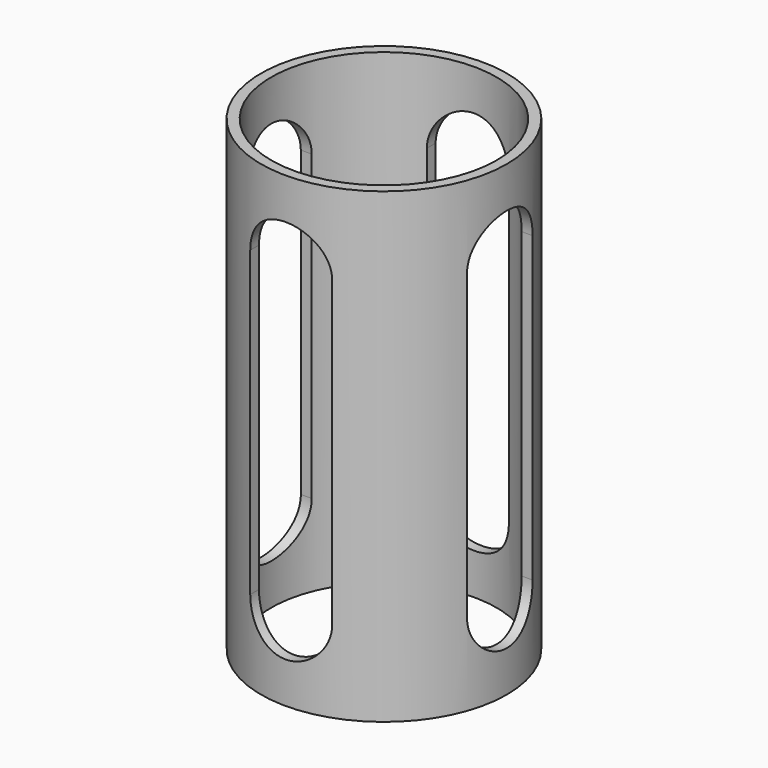
from build123d import *

# Parameters (mm, degrees)
F0_R            = 19.05
F0_R_2          = 17.4625
F1_DEPTH        = 72.39
F3_DEPTH        = 25.4
F3_COPIES_COUNT = 4


# Not quite as in the source:
# - a pattern or mirror of a feature is missing from the dataset's text; its kind, count and spacing are read off the source's solid


with BuildPart() as f1:
    # F0 (on Top) → F1 (new body)
    with BuildSketch(Plane.XY):
        Circle(F0_R)
        Circle(F0_R_2, mode=Mode.SUBTRACT)
    extrude(amount=F1_DEPTH)

    # F2 (on Front) → F3 (cut)
    with BuildSketch(Plane.XZ):
        with BuildLine():
            Line((-6.35, 59.69), (-6.35, 12.7))
            ThreePointArc((-6.35, 12.7), (0, 6.35), (6.35, 12.7))
            Line((6.35, 12.7), (6.35, 59.69))
            ThreePointArc((6.35, 59.69), (0, 66.04), (-6.35, 59.69))
        make_face()
    f3 = extrude(amount=-F3_DEPTH, mode=Mode.SUBTRACT)

    # F3_copies: F3 ×4 about axis
    f3_copies_axis = Axis((0, 0, 0), (0, 0, 1))
    for i in range(1, F3_COPIES_COUNT):
        add(f3.rotate(f3_copies_axis, i * 360 / F3_COPIES_COUNT), mode=Mode.SUBTRACT)


solid = f1.part
